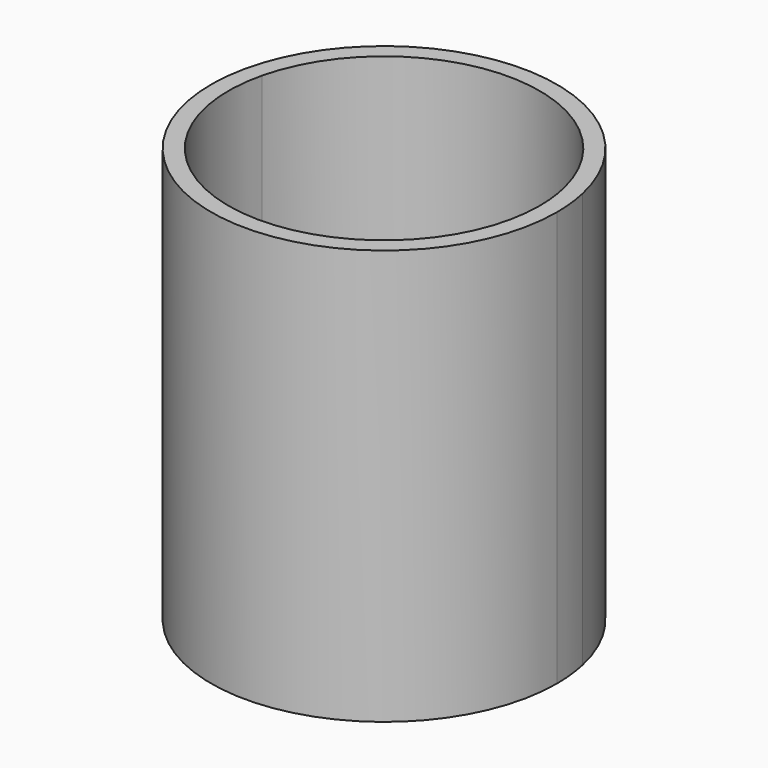
from build123d import *

# Parameters (mm, degrees)
F1_DEPTH       = 20
F2_DEPTH       = 4
F4_D           = 3.85
F4_CSINK_D     = 7.38
F4_CSINK_ANGLE = 90
F5_DEPTH       = 20


with BuildPart() as f1:
    # F0 (on Top) → F1 (new body)
    with BuildSketch(Plane.XY):
        with BuildLine():
            Line((8.745685, 2.124381), (9.771745, 2.124381))
            ThreePointArc((9.771745, 2.124381), (0, 10), (-9.771745, 2.124381))
            Line((-9.771745, 2.124381), (-8.745685, 2.124381))
            ThreePointArc((-8.745685, 2.124381), (0, 9), (8.745685, 2.124381))
        make_face()
    extrude(amount=F1_DEPTH)

    # F0 (on Top) → F2 (join)
    with BuildSketch(Plane.XY):
        with BuildLine():
            ThreePointArc((9, 0), (8.936195, 1.069775), (8.745685, 2.124381))
            Line((8.745685, 2.124381), (-8.745685, 2.124381))
            ThreePointArc((-8.745685, 2.124381), (-1.069775, -8.936195), (9, 0))
        make_face()
        with BuildLine():
            ThreePointArc((-9.771745, 2.124381), (-1.068304, -9.942773), (10, 0))
            ThreePointArc((10, 0), (9.942773, 1.068304), (9.771745, 2.124381))
            Line((9.771745, 2.124381), (8.745685, 2.124381))
            ThreePointArc((8.745685, 2.124381), (8.936195, 1.069775), (9, 0))
            ThreePointArc((9, 0), (-1.069775, -8.936195), (-8.745685, 2.124381))
            Line((-8.745685, 2.124381), (-9.771745, 2.124381))
        make_face()
        with BuildLine():
            Line((8.745685, 2.124381), (9.771745, 2.124381))
            ThreePointArc((9.771745, 2.124381), (0, 10), (-9.771745, 2.124381))
            Line((-9.771745, 2.124381), (-8.745685, 2.124381))
            ThreePointArc((-8.745685, 2.124381), (0, 9), (8.745685, 2.124381))
        make_face()
        with BuildLine():
            Line((-8.745685, 2.124381), (8.745685, 2.124381))
            ThreePointArc((8.745685, 2.124381), (0, 9), (-8.745685, 2.124381))
        make_face()
    extrude(amount=-F2_DEPTH)

    # F4 (through all)
    with Locations(Plane.XY):
        with Locations((0, 0)):
            CounterSinkHole(F4_D / 2, F4_CSINK_D / 2, counter_sink_angle=F4_CSINK_ANGLE)

    # F0 (on Top) → F5 (join)
    with BuildSketch(Plane.XY):
        with BuildLine():
            ThreePointArc((-9.771745, 2.124381), (-1.068304, -9.942773), (10, 0))
            ThreePointArc((10, 0), (9.942773, 1.068304), (9.771745, 2.124381))
            Line((9.771745, 2.124381), (8.745685, 2.124381))
            ThreePointArc((8.745685, 2.124381), (8.936195, 1.069775), (9, 0))
            ThreePointArc((9, 0), (-1.069775, -8.936195), (-8.745685, 2.124381))
            Line((-8.745685, 2.124381), (-9.771745, 2.124381))
        make_face()
    extrude(amount=F5_DEPTH)


solid = f1.part
